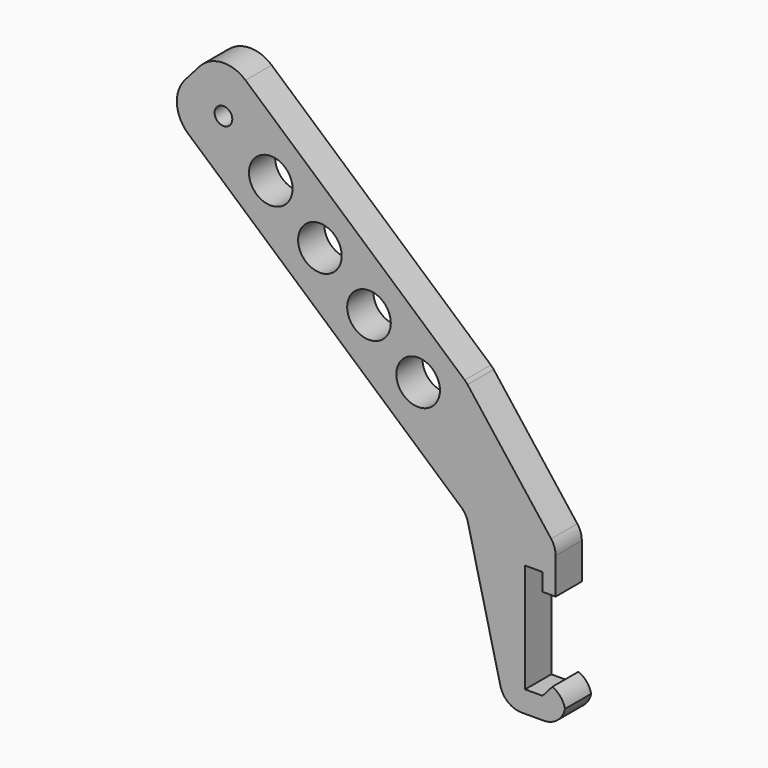
from build123d import *

# Parameters (mm, degrees)
F0_R         = 10
F1_DEPTH     = 15
F2_R         = 15
F3_T1_DEPTH  = 32.0168478214
F3_T3_DEPTH  = 19.855092474
F3_T5_DEPTH  = 60.8257569496
F3_T7_DEPTH  = 65
F3_T9_DEPTH  = 54.2875458035
F3_T11_DEPTH = 15
F5_R         = 12
F6_DEPTH     = 12
F7_R         = 11.99999
F8_R         = 4.05
F9_DEPTH     = 27.001


# Not quite as in the source:
# - a fillet or chamfer that OpenCascade refuses, or shapes differently, is made with other operations: its cross-section is extruded or revolved along the edge and cut away or added
# - a fillet or chamfer is up to 0.001 mm smaller than in the source, because OpenCascade refuses the exact size


with BuildPart() as f1:
    # F0 (on Front) → F1 (new body)
    with BuildSketch(Plane.XZ):
        Polygon((-138.9475274131, 122.1416580278), (0, 0), (17.5, -71.8808303125), (45.5, -71.8808303125), (45.5, -56.8808303125), (39.5, -56.8808303125), (35, -62), (27, -62), (27, -12), (35, -12), (35, -20), (41, -20), (41, 0), (0, 53.2575148171), (-112.5385202719, 152.1843666577), align=None)
        with Locations((-67.1597420143, 85.6654484175)):
            Circle(F0_R, mode=Mode.SUBTRACT)
        with Locations((-89.6917734867, 105.4722037734)):
            Circle(F0_R, mode=Mode.SUBTRACT)
        with Locations((-44.6277105419, 65.8586930616)):
            Circle(F0_R, mode=Mode.SUBTRACT)
        with Locations((-22.0956790695, 46.0519377058)):
            Circle(F0_R, mode=Mode.SUBTRACT)
    extrude(amount=F1_DEPTH)

    # F2
    f2_edges = [f1.edges().sort_by_distance(p)[0] for p in [
        (-112.53852, -7.5, 152.184367),
        (-138.947527, -7.5, 122.141658),
    ]]
    fillet(f2_edges, radius=F2_R)

    # F3: fillet of radius 10 on 6 edges, made by hand

    # F3_s2 → F3_t1 (cut)
    with BuildSketch(Plane.XZ.offset(-8.5084239107)):
        with BuildLine():
            ThreePointArc((38.9238894384, 2.6967924145), (40.4667548395, -0.1814830349), (41, -3.4033695643))
            Line((41, -3.4033695643), (41.2, -3.4033695643))
            Line((41.2, -3.4033695643), (41.2, 0.0680673913))
            Line((41.2, 0.0680673913), (39.0823672272, 2.8187956541))
            Line((39.0823672272, 2.8187956541), (38.9238894384, 2.6967924145))
        make_face()
    extrude(amount=F3_T1_DEPTH, mode=Mode.SUBTRACT)

    # F3_s4 → F3_t3 (cut)
    with BuildSketch(Plane.XZ.offset(-2.427546237)):
        with BuildLine():
            ThreePointArc((-0.7293006428, 53.8986056762), (-0.0343212423, 53.2253561798), (0.5923370103, 52.4880904975))
            Line((0.5923370103, 52.4880904975), (0.750814799, 52.6100937371))
            Line((0.750814799, 52.6100937371), (0.1466310486, 53.3949065431))
            Line((0.1466310486, 53.3949065431), (-0.5972556071, 54.0488192193))
            Line((-0.5972556071, 54.0488192193), (-0.7293006428, 53.8986056762))
        make_face()
    extrude(amount=F3_T3_DEPTH, mode=Mode.SUBTRACT)

    # F3_s6 → F3_t5 (cut)
    with BuildSketch(Plane.XZ.offset(-22.9128784748)):
        with BuildLine():
            ThreePointArc((45.5, -66.0459817024), (43.8666002653, -60.5687561273), (39.5, -56.8808303125))
            Line((39.5, -56.8808303125), (39.58, -56.6975272847))
            ThreePointArc((39.58, -56.6975272847), (42.5, -56.6808303125), (45.5, -56.6808303125))
            Line((45.5, -56.6808303125), (45.7, -56.8808303125))
            Line((45.7, -56.8808303125), (45.7, -66.0459817024))
            Line((45.7, -66.0459817024), (45.5, -66.0459817024))
        make_face()
    extrude(amount=F3_T5_DEPTH, mode=Mode.SUBTRACT)

    # F3_s8 → F3_t7 (cut)
    with BuildSketch(Plane.XZ.offset(-25)):
        with BuildLine():
            ThreePointArc((35.5, -71.8808303125), (42.5710678119, -68.9518981244), (45.5, -61.8808303125))
            Line((45.5, -61.8808303125), (45.7, -61.8808303125))
            Line((45.7, -61.8808303125), (45.7, -72.0808303125))
            Line((45.7, -72.0808303125), (35.5, -72.0808303125))
            Line((35.5, -72.0808303125), (35.5, -71.8808303125))
        make_face()
    extrude(amount=F3_T7_DEPTH, mode=Mode.SUBTRACT)

    # F3_s10 → F3_t9 (cut)
    with BuildSketch(Plane.XZ.offset(-19.6437729018)):
        with BuildLine():
            ThreePointArc((15.6413136753, -64.2463208091), (19.1791155574, -69.7438737743), (25.3575091607, -71.8808303125))
            Line((25.3575091607, -71.8808303125), (25.3575091607, -72.0808303125))
            Line((25.3575091607, -72.0808303125), (17.3428498168, -72.0808303125))
            Line((17.3428498168, -72.0808303125), (15.4469897656, -64.2936306191))
            Line((15.4469897656, -64.2936306191), (15.6413136753, -64.2463208091))
        make_face()
    extrude(amount=F3_T9_DEPTH, mode=Mode.SUBTRACT)

    # F3_s12 → F3_t11 (join)
    with BuildSketch(Plane.XZ):
        with BuildLine():
            ThreePointArc((-2.3681074114, 2.0816819918), (-0.4151755765, -0.2512704506), (0.7458362887, -3.0635046691))
            Line((0.7458362887, -3.0635046691), (0.9401601984, -3.0161948591))
            Line((0.9401601984, -3.0161948591), (0.1794071839, 0.1085799033))
            Line((0.1794071839, 0.1085799033), (-2.2360623757, 2.2318955349))
            Line((-2.2360623757, 2.2318955349), (-2.3681074114, 2.0816819918))
        make_face()
    extrude(amount=F3_T11_DEPTH)

    # F5 (on face) → F6 (join)
    with BuildSketch(Plane(origin=(0, 0, 0), x_dir=(-1, 0, 0), z_dir=(0, 1, 0))):
        with Locations((111.3978201201, 124.552878143)):
            Circle(F5_R)
    extrude(amount=F6_DEPTH)

    # F7 (radius 12 in the source; OpenCascade refuses exactly that, so slightly less here)
    f7_edges = [f1.edges().sort_by_distance(p)[0] for p in [
        (-99.39782, 12, 124.552878),
    ]]
    fillet(f7_edges, radius=F7_R)

    # F8 (on face) → F9 (cut, through all)
    with BuildSketch(Plane.XZ.offset(15)):
        with Locations((-111.3978201201, 124.552878143)):
            Circle(F8_R)
    extrude(amount=-F9_DEPTH, mode=Mode.SUBTRACT)


solid = f1.part
